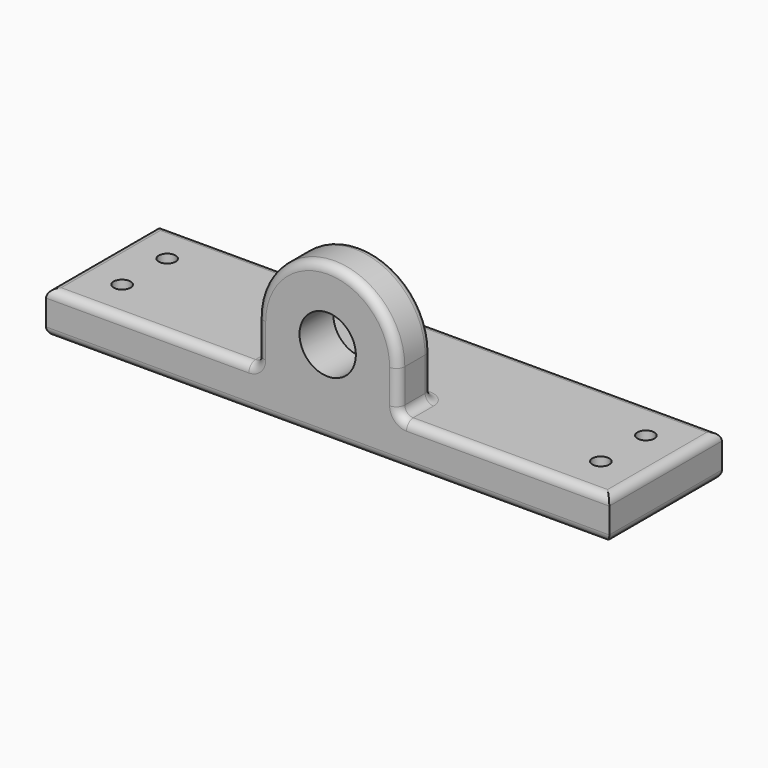
from build123d import *

# Parameters (mm, degrees)
F0_W     = 200
F0_H     = 50
F1_DEPTH = 15
F3_DEPTH = 15
F4_R     = 3
F5_DEPTH = 15.001
F6_R     = 3


with BuildPart() as f1:
    # F0 (on Top) → F1 (new body)
    with BuildSketch(Plane.XY):
        Rectangle(F0_W, F0_H)
    extrude(amount=F1_DEPTH)

    # F2 (on face) → F3 (join)
    with BuildSketch(Plane.XZ.offset(25)):
        with BuildLine():
            Line((25, 15), (20, 15))
            ThreePointArc((20, 15), (0, 5), (-20, 15))
            Line((-20, 15), (-25, 15))
            Line((-25, 15), (-25, 0))
            Line((-25, 0), (25, 0))
            Line((25, 0), (25, 15))
        make_face()
        with BuildLine():
            ThreePointArc((-20, 15), (-23.7170824513, 22.0943058496), (-25, 30))
            Line((-25, 30), (-25, 15))
            Line((-25, 15), (-20, 15))
        make_face()
        with BuildLine():
            Line((25, 15), (25, 30))
            ThreePointArc((25, 30), (23.7170824513, 22.0943058496), (20, 15))
            Line((20, 15), (25, 15))
        make_face()
        with BuildLine():
            ThreePointArc((-20, 15), (0, 5), (20, 15))
            Line((20, 15), (-20, 15))
        make_face()
        with BuildLine():
            ThreePointArc((20, 15), (23.7170824513, 22.0943058496), (25, 30))
            Line((25, 30), (10, 30))
            ThreePointArc((10, 30), (0, 20), (-10, 30))
            Line((-10, 30), (-25, 30))
            ThreePointArc((-25, 30), (-23.7170824513, 22.0943058496), (-20, 15))
            Line((-20, 15), (20, 15))
        make_face()
        with BuildLine():
            Line((10, 30), (25, 30))
            ThreePointArc((25, 30), (0, 55), (-25, 30))
            Line((-25, 30), (-10, 30))
            ThreePointArc((-10, 30), (0, 40), (10, 30))
        make_face()
    extrude(amount=-F3_DEPTH)

    # F4 (on face) → F5 (cut, through all)
    with BuildSketch(Plane.XY.offset(15)):
        with Locations((-85, 10)):
            Circle(F4_R)
        with Locations((-85, -10)):
            Circle(F4_R)
        with Locations((85, 10)):
            Circle(F4_R)
        with Locations((85, -10)):
            Circle(F4_R)
    extrude(amount=-F5_DEPTH, mode=Mode.SUBTRACT)

    # F6
    f6_edges = [f1.edges().sort_by_distance(p)[0] for p in [
        (-62.5, -25, 15),
        (-100, 0, 15),
        (0, 25, 15),
        (100, 0, 15),
        (62.5, -25, 15),
        (25, -17.5, 15),
        (-25, -17.5, 15),
        (-25, -10, 22.5),
        (0, -25, 0),
        (100, 0, 0),
        (0, 25, 0),
        (-100, 0, 0),
        (-25, -25, 22.5),
        (0, -25, 55),
        (25, -25, 22.5),
        (0, -10, 15),
        (0, -10, 55),
        (25, -10, 22.5),
    ]]
    fillet(f6_edges, radius=F6_R)


solid = f1.part
